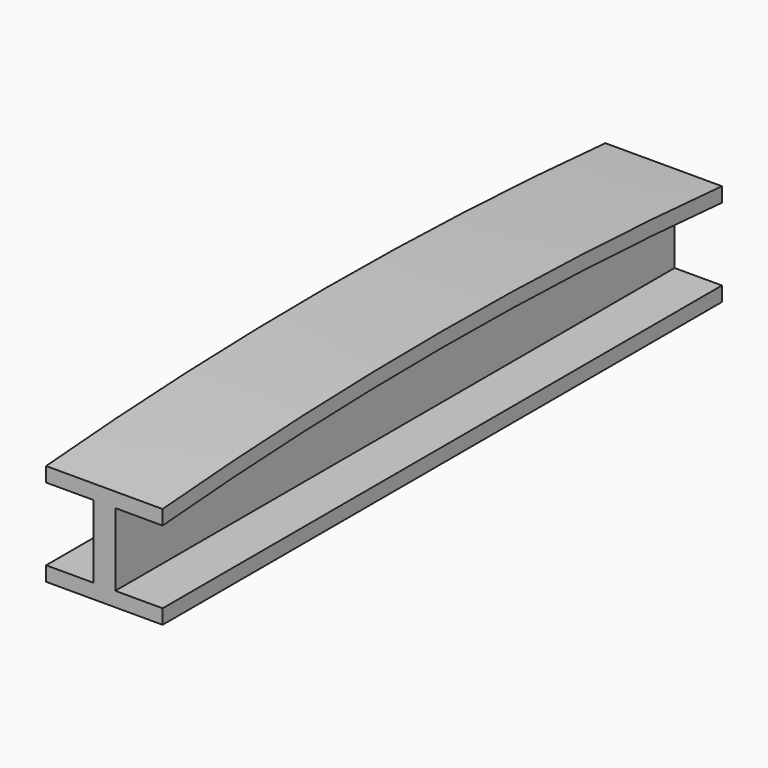
from build123d import *

# Parameters (mm, degrees)
F0_W     = 304.8
F0_H     = 6.35
F1_DEPTH = 50.8
F3_DEPTH = 0.8125
F5_DEPTH = 20.6502


# Not quite as in the source:
# - a pattern or mirror of a feature is missing from the dataset's text; its kind, count and spacing are read off the source's solid


with BuildPart() as f1:
    # F0 (on Right) → F1 (new body)
    with BuildSketch(Plane.YZ):
        with BuildLine():
            Line((-304.8, 6.35), (0, 6.35))
            Line((0, 6.35), (0, 38.1))
            ThreePointArc((0, 38.1), (-152.4, 44.45), (-304.8, 38.1))
            Line((-304.8, 38.1), (-304.8, 6.35))
        make_face()
        with BuildLine():
            ThreePointArc((-304.8, 38.1), (-152.4, 44.45), (0, 38.1))
            Line((0, 38.1), (0, 44.45))
            ThreePointArc((0, 44.45), (-152.4, 50.8), (-304.8, 44.45))
            Line((-304.8, 44.45), (-304.8, 38.1))
        make_face()
        with Locations((-152.4, 3.175)):
            Rectangle(F0_W, F0_H)
    extrude(amount=F1_DEPTH)

    # F2 (on face) → F3 (cut)
    with BuildSketch(Plane.YZ.offset(50.8)):
        with BuildLine():
            Line((0, 6.35), (0, 38.1))
            ThreePointArc((0, 38.1), (-152.4, 44.45), (-304.8, 38.1))
            Line((-304.8, 38.1), (-304.8, 6.35))
            Line((-304.8, 6.35), (0, 6.35))
        make_face()
    extrude(amount=-F3_DEPTH, mode=Mode.SUBTRACT)

    # F4 (on face) → F5 (cut)
    with BuildSketch(Plane(origin=(0, 0, 0), x_dir=(0, -1, 0), z_dir=(-1, 0, 0))):
        with BuildLine():
            Line((304.8, 6.35), (304.8, 38.1))
            ThreePointArc((304.8, 38.1), (152.4, 44.45), (0, 38.1))
            Line((0, 38.1), (0, 6.35))
            Line((0, 6.35), (304.8, 6.35))
        make_face()
    f5 = extrude(amount=-F5_DEPTH, mode=Mode.SUBTRACT)

    # F5_copies: F5 across plane
    add(f5.mirror(Plane(origin=(25.40635, 0, 0), x_dir=(0, 0, 1), z_dir=(1, 0, 0))), mode=Mode.SUBTRACT)


solid = f1.part
